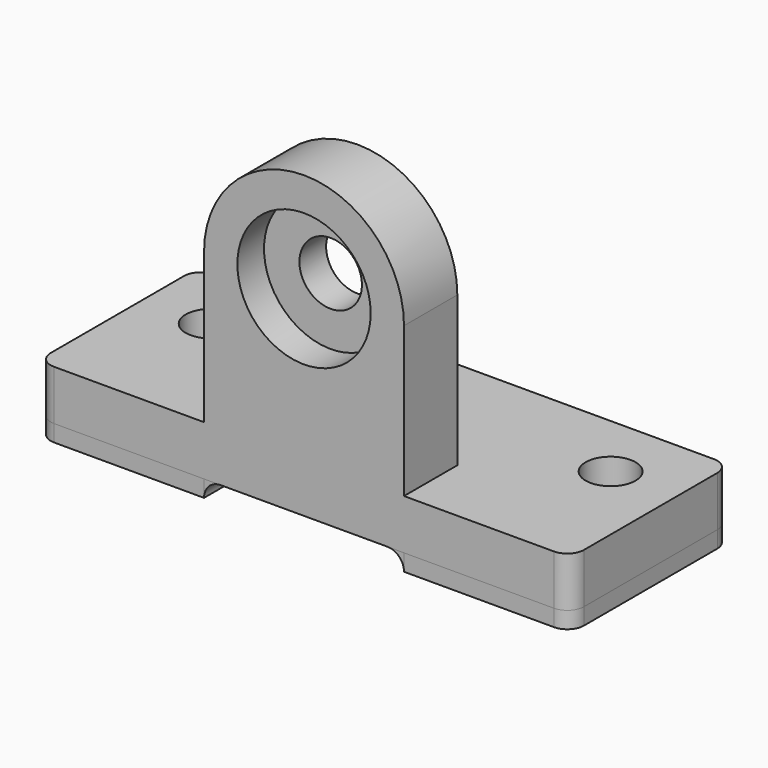
from build123d import *

# Parameters (mm, degrees)
F0_W           = 101.6
F0_H           = 38.1
F1_DEPTH       = 9.525
F3_DEPTH       = 12.7
F5_D           = 11.90625
F5_CBORE_D     = 25.4
F5_CBORE_DEPTH = 6.35
F7_W           = 31.75
F7_H           = 3.175
F8_DEPTH       = 38.1
F10_D          = 9.525
F10_2_D        = 9.525
F10_3_D        = 9.525
F11_R          = 3.175
F11_2_R        = 3.175
F11_3_R        = 3.175
F13_DEPTH      = 38.1


# Not quite as in the source:
# - a length typed as a fraction of an inch, garbled in the dataset ("3 / 203.2 mm" for 3/8 in), is restored


with BuildPart() as f1:
    # F0 (on Top) → F1 (new body)
    with BuildSketch(Plane.XY):
        with Locations((50.8, 19.05)):
            Rectangle(F0_W, F0_H)
    extrude(amount=F1_DEPTH)

    # F2 (on face) → F3 (join)
    with BuildSketch(Plane.XZ):
        with BuildLine():
            Line((31.75, 38.1), (31.75, 0))
            Line((31.75, 0), (69.85, 0))
            Line((69.85, 0), (69.85, 38.1))
            ThreePointArc((69.85, 38.1), (50.8, 57.15), (31.75, 38.1))
        make_face()
    extrude(amount=-F3_DEPTH)

    # F5 (through all)
    with Locations(Plane.XZ):
        with Locations((50.8, 38.1)):
            CounterBoreHole(F5_D / 2, F5_CBORE_D / 2, F5_CBORE_DEPTH)

    # F10 (through all)
    with Locations(Plane.XY.offset(9.525)):
        with Locations((12.7, 25.4), (88.9, 25.4)):
            Hole(F10_D / 2)

    # F11
    f11_edges = [f1.edges().sort_by_distance(p)[0] for p in [
        (0, 0, 4.7625),
        (0, 38.1, 4.7625),
        (101.6, 0, 4.7625),
        (101.6, 38.1, 4.7625),
    ]]
    fillet(f11_edges, radius=F11_R)


with BuildPart() as f8:
    # F7 (on face) → F8 (new body, through all)
    with BuildSketch(Plane.XZ):
        with Locations((15.875, -1.5875)):
            Rectangle(F7_W, F7_H)
    extrude(amount=-F8_DEPTH)

    # F10#2 (through all)
    with Locations(Plane.XY.offset(9.525)):
        with Locations((12.7, 25.4), (88.9, 25.4)):
            Hole(F10_2_D / 2)

    # F11#2
    f11_2_edges = [f8.edges().sort_by_distance(p)[0] for p in [
        (0, 0, -1.5875),
        (0, 38.1, -1.5875),
    ]]
    fillet(f11_2_edges, radius=F11_2_R)


with BuildPart() as f8b:
    # F7 (on face) → F8, piece 2 (new body, through all)
    with BuildSketch(Plane.XZ):
        with Locations((85.725, -1.5875)):
            Rectangle(F7_W, F7_H)
    extrude(amount=-F8_DEPTH)

    # F10#3 (through all)
    with Locations(Plane.XY.offset(9.525)):
        with Locations((12.7, 25.4), (88.9, 25.4)):
            Hole(F10_3_D / 2)

    # F11#3
    f11_3_edges = [f8b.edges().sort_by_distance(p)[0] for p in [
        (101.6, 0, -1.5875),
        (101.6, 38.1, -1.5875),
    ]]
    fillet(f11_3_edges, radius=F11_3_R)


with BuildPart() as f13:
    # F12 (on face) → F13 (new body, through all)
    with BuildSketch(Plane(origin=(0, 38.1, 0), x_dir=(-1, 0, 0), z_dir=(0, 1, 0))):
        with BuildLine():
            Line((-31.7329987884, 0), (-34.925, 0))
            ThreePointArc((-34.925, 0), (-32.6799359697, -0.9299359697), (-31.75, -3.175))
            Line((-31.75, -3.175), (-31.7329987884, 0))
        make_face()
    extrude(amount=-F13_DEPTH)


with BuildPart() as f13b:
    # F12 (on face) → F13, piece 2 (new body, through all)
    with BuildSketch(Plane(origin=(0, 38.1, 0), x_dir=(-1, 0, 0), z_dir=(0, 1, 0))):
        with BuildLine():
            Line((-69.85, 0), (-69.85, -3.175))
            ThreePointArc((-69.85, -3.175), (-68.9200640303, -0.9299359697), (-66.675, 0))
            Line((-66.675, 0), (-69.85, 0))
        make_face()
    extrude(amount=-F13_DEPTH)


solid = Compound([f1.part, f8.part, f8b.part, f13.part, f13b.part])
